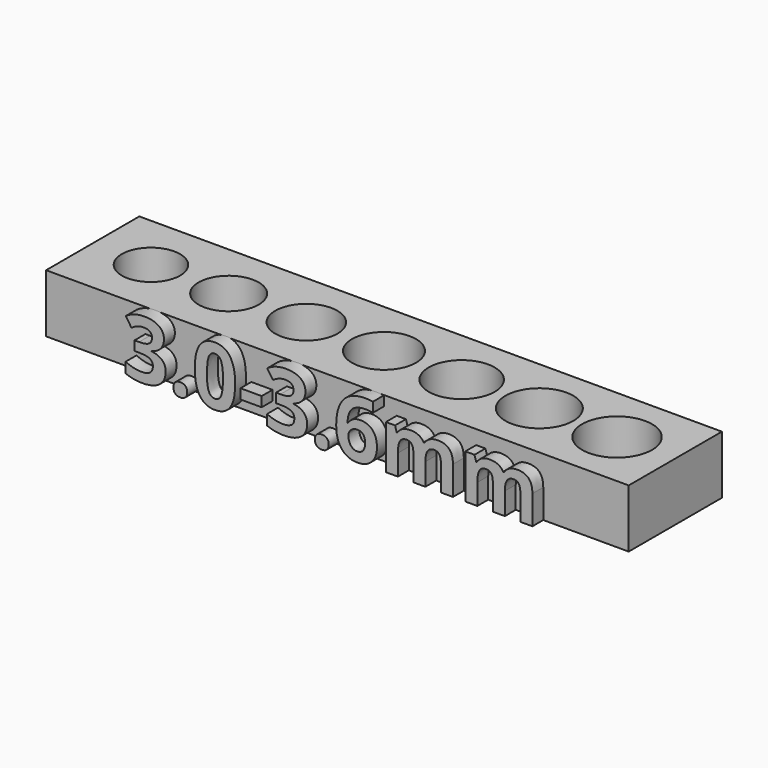
from build123d import *

# Parameters (mm, degrees)
F0_W         = 30
F0_H         = 6
F0_R         = 1.5
F0_R_2       = 1.55
F0_R_3       = 1.6
F0_R_4       = 1.65
F0_R_5       = 1.7
F0_R_6       = 1.75
F0_R_7       = 1.8
F1_DEPTH     = 3
F2_TEXT_SIZE = 4.1666666667
F3_DEPTH     = 0.7


# Not quite as in the source:
# - Text() gives the source's letters only with a copy of the font that has no kerning and outlines rounded to 1/6400 em; it was checked with that copy


with BuildPart() as f1:
    # F0 (on Top) → F1 (new body)
    with BuildSketch(Plane.XY):
        Rectangle(F0_W, F0_H)
        with Locations((-12, 0)):
            Circle(F0_R, mode=Mode.SUBTRACT)
        with Locations((-8, 0)):
            Circle(F0_R_2, mode=Mode.SUBTRACT)
        with Locations((-4, 0)):
            Circle(F0_R_3, mode=Mode.SUBTRACT)
        Circle(F0_R_4, mode=Mode.SUBTRACT)
        with Locations((4, 0)):
            Circle(F0_R_5, mode=Mode.SUBTRACT)
        with Locations((8, 0)):
            Circle(F0_R_6, mode=Mode.SUBTRACT)
        with Locations((12, 0)):
            Circle(F0_R_7, mode=Mode.SUBTRACT)
    extrude(amount=F1_DEPTH)

    # F2 (on face) → F3 (join)
    with BuildSketch(Plane.XZ.offset(3)):
        with Locations((-10.5, 0)):
            Text('3.0-3.6mm', F2_TEXT_SIZE, font='Open Sans', font_style=FontStyle.BOLD, text_align=(TextAlign.LEFT, TextAlign.BOTTOM))
    extrude(amount=F3_DEPTH)


solid = f1.part
